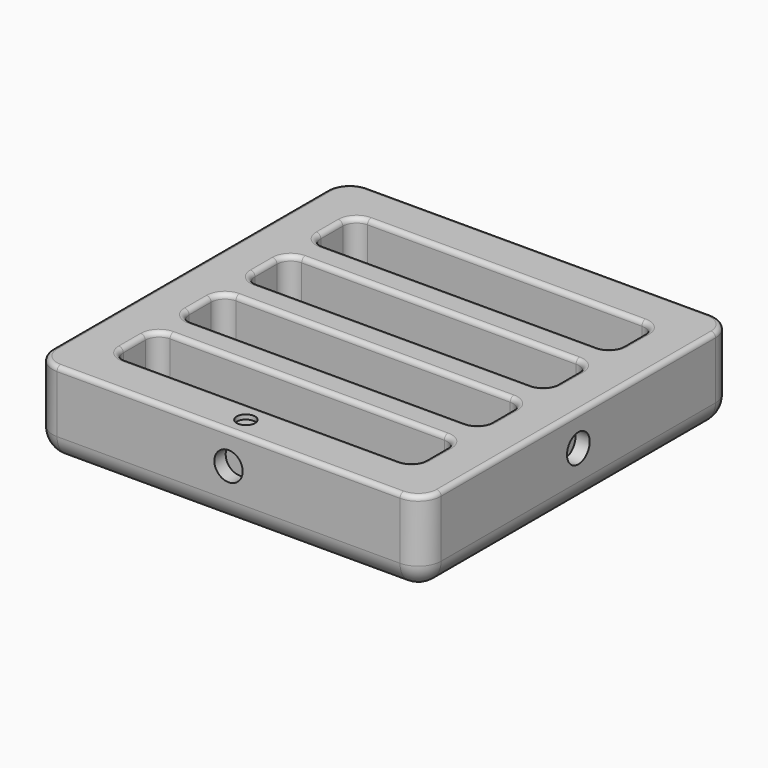
from build123d import *

# Parameters (mm, degrees)
F0_W      = 85
F0_H      = 85
F0_R      = 2
F3_DEPTH  = 18.5
F4_DEPTH  = 14
F5_R      = 5
F6_R      = 3
F7_R      = 1
F8_R      = 3.1
F9_DEPTH  = 3.1
F10_R     = 3.1
F11_DEPTH = 3.1
F12_R     = 3.1
F13_DEPTH = 3.1
F14_R     = 3.1
F15_DEPTH = 3.1
F16_DEPTH = 1
F17_ANGLE = 180


# Not quite as in the source:
# - a feature names something its author has since deleted; it is built from what else it names


with BuildPart() as f3:
    # F0 (on Top) → F3 (new body)
    with BuildSketch(Plane.XY):
        Rectangle(F0_W, F0_H)
        with Locations((0, -37.75)):
            Circle(F0_R, mode=Mode.SUBTRACT)
        with BuildLine():
            Line((-33, -30), (-33, -24))
            ThreePointArc((-33, -24), (-32.1213203436, -21.8786796564), (-30, -21))
            Line((-30, -21), (30, -21))
            ThreePointArc((30, -21), (32.1213203436, -21.8786796564), (33, -24))
            Line((33, -24), (33, -30))
            ThreePointArc((33, -30), (32.1213203436, -32.1213203436), (30, -33))
            Line((30, -33), (-30, -33))
            ThreePointArc((-30, -33), (-32.1213203436, -32.1213203436), (-33, -30))
        make_face(mode=Mode.SUBTRACT)
        with BuildLine():
            Line((-33, -12), (-33, -6))
            ThreePointArc((-33, -6), (-32.1213203436, -3.8786796564), (-30, -3))
            Line((-30, -3), (30, -3))
            ThreePointArc((30, -3), (32.1213203436, -3.8786796564), (33, -6))
            Line((33, -6), (33, -12))
            ThreePointArc((33, -12), (32.1213203436, -14.1213203436), (30, -15))
            Line((30, -15), (-30, -15))
            ThreePointArc((-30, -15), (-32.1213203436, -14.1213203436), (-33, -12))
        make_face(mode=Mode.SUBTRACT)
        with BuildLine():
            Line((-33, 6), (-33, 12))
            ThreePointArc((-33, 12), (-32.1213203436, 14.1213203436), (-30, 15))
            Line((-30, 15), (30, 15))
            ThreePointArc((30, 15), (32.1213203436, 14.1213203436), (33, 12))
            Line((33, 12), (33, 6))
            ThreePointArc((33, 6), (32.1213203436, 3.8786796564), (30, 3))
            Line((30, 3), (-30, 3))
            ThreePointArc((-30, 3), (-32.1213203436, 3.8786796564), (-33, 6))
        make_face(mode=Mode.SUBTRACT)
        with BuildLine():
            ThreePointArc((-33, 30), (-32.1213203436, 32.1213203436), (-30, 33))
            Line((-30, 33), (30, 33))
            ThreePointArc((30, 33), (32.1213203436, 32.1213203436), (33, 30))
            Line((33, 30), (33, 24))
            ThreePointArc((33, 24), (32.1213203436, 21.8786796564), (30, 21))
            Line((30, 21), (-30, 21))
            ThreePointArc((-30, 21), (-32.1213203436, 21.8786796564), (-33, 24))
            Line((-33, 24), (-33, 30))
        make_face(mode=Mode.SUBTRACT)
        with BuildLine():
            Line((30, 33), (-30, 33))
            ThreePointArc((-30, 33), (-32.1213203436, 32.1213203436), (-33, 30))
            Line((-33, 30), (-33, 24))
            ThreePointArc((-33, 24), (-32.1213203436, 21.8786796564), (-30, 21))
            Line((-30, 21), (30, 21))
            ThreePointArc((30, 21), (32.1213203436, 21.8786796564), (33, 24))
            Line((33, 24), (33, 30))
            ThreePointArc((33, 30), (32.1213203436, 32.1213203436), (30, 33))
        make_face()
        with BuildLine():
            ThreePointArc((-30, 15), (-32.1213203436, 14.1213203436), (-33, 12))
            Line((-33, 12), (-33, 6))
            ThreePointArc((-33, 6), (-32.1213203436, 3.8786796564), (-30, 3))
            Line((-30, 3), (30, 3))
            ThreePointArc((30, 3), (32.1213203436, 3.8786796564), (33, 6))
            Line((33, 6), (33, 12))
            ThreePointArc((33, 12), (32.1213203436, 14.1213203436), (30, 15))
            Line((30, 15), (-30, 15))
        make_face()
        with BuildLine():
            ThreePointArc((-30, -3), (-32.1213203436, -3.8786796564), (-33, -6))
            Line((-33, -6), (-33, -12))
            ThreePointArc((-33, -12), (-32.1213203436, -14.1213203436), (-30, -15))
            Line((-30, -15), (30, -15))
            ThreePointArc((30, -15), (32.1213203436, -14.1213203436), (33, -12))
            Line((33, -12), (33, -6))
            ThreePointArc((33, -6), (32.1213203436, -3.8786796564), (30, -3))
            Line((30, -3), (-30, -3))
        make_face()
        with BuildLine():
            ThreePointArc((-30, -21), (-32.1213203436, -21.8786796564), (-33, -24))
            Line((-33, -24), (-33, -30))
            ThreePointArc((-33, -30), (-32.1213203436, -32.1213203436), (-30, -33))
            Line((-30, -33), (30, -33))
            ThreePointArc((30, -33), (32.1213203436, -32.1213203436), (33, -30))
            Line((33, -30), (33, -24))
            ThreePointArc((33, -24), (32.1213203436, -21.8786796564), (30, -21))
            Line((30, -21), (-30, -21))
        make_face()
        with Locations((0, -37.75)):
            Circle(F0_R)
    extrude(amount=F3_DEPTH)

    # F0 (on Top) → F4 (cut)
    with BuildSketch(Plane.XY):
        with BuildLine():
            Line((30, 33), (-30, 33))
            ThreePointArc((-30, 33), (-32.1213203436, 32.1213203436), (-33, 30))
            Line((-33, 30), (-33, 24))
            ThreePointArc((-33, 24), (-32.1213203436, 21.8786796564), (-30, 21))
            Line((-30, 21), (30, 21))
            ThreePointArc((30, 21), (32.1213203436, 21.8786796564), (33, 24))
            Line((33, 24), (33, 30))
            ThreePointArc((33, 30), (32.1213203436, 32.1213203436), (30, 33))
        make_face()
        with BuildLine():
            ThreePointArc((-30, 15), (-32.1213203436, 14.1213203436), (-33, 12))
            Line((-33, 12), (-33, 6))
            ThreePointArc((-33, 6), (-32.1213203436, 3.8786796564), (-30, 3))
            Line((-30, 3), (30, 3))
            ThreePointArc((30, 3), (32.1213203436, 3.8786796564), (33, 6))
            Line((33, 6), (33, 12))
            ThreePointArc((33, 12), (32.1213203436, 14.1213203436), (30, 15))
            Line((30, 15), (-30, 15))
        make_face()
        with BuildLine():
            ThreePointArc((-30, -3), (-32.1213203436, -3.8786796564), (-33, -6))
            Line((-33, -6), (-33, -12))
            ThreePointArc((-33, -12), (-32.1213203436, -14.1213203436), (-30, -15))
            Line((-30, -15), (30, -15))
            ThreePointArc((30, -15), (32.1213203436, -14.1213203436), (33, -12))
            Line((33, -12), (33, -6))
            ThreePointArc((33, -6), (32.1213203436, -3.8786796564), (30, -3))
            Line((30, -3), (-30, -3))
        make_face()
        with BuildLine():
            ThreePointArc((-30, -21), (-32.1213203436, -21.8786796564), (-33, -24))
            Line((-33, -24), (-33, -30))
            ThreePointArc((-33, -30), (-32.1213203436, -32.1213203436), (-30, -33))
            Line((-30, -33), (30, -33))
            ThreePointArc((30, -33), (32.1213203436, -32.1213203436), (33, -30))
            Line((33, -30), (33, -24))
            ThreePointArc((33, -24), (32.1213203436, -21.8786796564), (30, -21))
            Line((30, -21), (-30, -21))
        make_face()
    extrude(amount=F4_DEPTH, mode=Mode.SUBTRACT)

    # F5
    f5_edges = [f3.edges().sort_by_distance(p)[0] for p in [
        (0, 42.5, 18.5),
        (-42.5, 0, 18.5),
        (0, -42.5, 18.5),
        (42.5, 0, 18.5),
        (42.5, 42.5, 9.25),
        (-42.5, 42.5, 9.25),
        (-42.5, -42.5, 9.25),
        (42.5, -42.5, 9.25),
    ]]
    fillet(f5_edges, radius=F5_R)

    # F6
    f6_edges = [f3.edges().sort_by_distance(p)[0] for p in [
        (0, 33, 14),
        (-32.12132, 32.12132, 14),
        (-33, 27, 14),
        (-32.12132, 21.87868, 14),
        (0, 21, 14),
        (32.12132, 21.87868, 14),
        (33, 27, 14),
        (32.12132, 32.12132, 14),
        (-32.12132, 14.12132, 14),
        (-33, 9, 14),
        (-32.12132, 3.87868, 14),
        (0, 3, 14),
        (32.12132, 3.87868, 14),
        (33, 9, 14),
        (32.12132, 14.12132, 14),
        (0, 15, 14),
        (-32.12132, -3.87868, 14),
        (-33, -9, 14),
        (-32.12132, -14.12132, 14),
        (0, -15, 14),
        (32.12132, -14.12132, 14),
        (33, -9, 14),
        (32.12132, -3.87868, 14),
        (0, -3, 14),
        (-32.12132, -21.87868, 14),
        (-33, -27, 14),
        (-32.12132, -32.12132, 14),
        (0, -33, 14),
        (32.12132, -32.12132, 14),
        (33, -27, 14),
        (32.12132, -21.87868, 14),
        (0, -21, 14),
    ]]
    fillet(f6_edges, radius=F6_R)

    # F7
    f7_edges = [f3.edges().sort_by_distance(p)[0] for p in [
        (0, 42.5, 0),
        (41.035534, 41.035534, 0),
        (-41.035534, 41.035534, 0),
        (42.5, 0, 0),
        (-42.5, 0, 0),
        (41.035534, -41.035534, 0),
        (-41.035534, -41.035534, 0),
        (0, -42.5, 0),
        (-32.12132, -21.87868, 0),
        (-33, -27, 0),
        (-32.12132, -32.12132, 0),
        (0, -33, 0),
        (32.12132, -32.12132, 0),
        (33, -27, 0),
        (32.12132, -21.87868, 0),
        (0, -21, 0),
        (-32.12132, -3.87868, 0),
        (-33, -9, 0),
        (-32.12132, -14.12132, 0),
        (0, -15, 0),
        (32.12132, -14.12132, 0),
        (33, -9, 0),
        (32.12132, -3.87868, 0),
        (0, -3, 0),
        (-32.12132, 14.12132, 0),
        (-33, 9, 0),
        (-32.12132, 3.87868, 0),
        (0, 3, 0),
        (32.12132, 3.87868, 0),
        (33, 9, 0),
        (32.12132, 14.12132, 0),
        (0, 15, 0),
        (0, 33, 0),
        (-32.12132, 32.12132, 0),
        (-33, 27, 0),
        (-32.12132, 21.87868, 0),
        (0, 21, 0),
        (32.12132, 21.87868, 0),
        (33, 27, 0),
        (32.12132, 32.12132, 0),
    ]]
    fillet(f7_edges, radius=F7_R)

    # F8 (on face) → F9 (cut)
    with BuildSketch(Plane.XZ.offset(42.5)):
        with Locations((0, 7)):
            Circle(F8_R)
    extrude(amount=-F9_DEPTH, mode=Mode.SUBTRACT)

    # F10 (on face) → F11 (cut)
    with BuildSketch(Plane(origin=(0, 42.5, 0), x_dir=(-1, 0, 0), z_dir=(0, 1, 0))):
        with Locations((0, 7)):
            Circle(F10_R)
    extrude(amount=-F11_DEPTH, mode=Mode.SUBTRACT)

    # F12 (on face) → F13 (cut)
    with BuildSketch(Plane(origin=(-42.5, 0, 0), x_dir=(0, -1, 0), z_dir=(-1, 0, 0))):
        with Locations((0, 7)):
            Circle(F12_R)
    extrude(amount=-F13_DEPTH, mode=Mode.SUBTRACT)

    # F14 (on face) → F15 (cut)
    with BuildSketch(Plane.YZ.offset(42.5)):
        with Locations((0, 7)):
            Circle(F14_R)
    extrude(amount=-F15_DEPTH, mode=Mode.SUBTRACT)

    # F0 (on Top) → F16 (cut)
    with BuildSketch(Plane.XY):
        with Locations((0, -37.75)):
            Circle(F0_R)
    extrude(amount=F16_DEPTH, mode=Mode.SUBTRACT)


with BuildPart() as f3_1:
    # F17: moved
    add(f3.part.rotate(Axis((0, 0, 0), (0, 1, 0)), F17_ANGLE))


solid = f3_1.part
